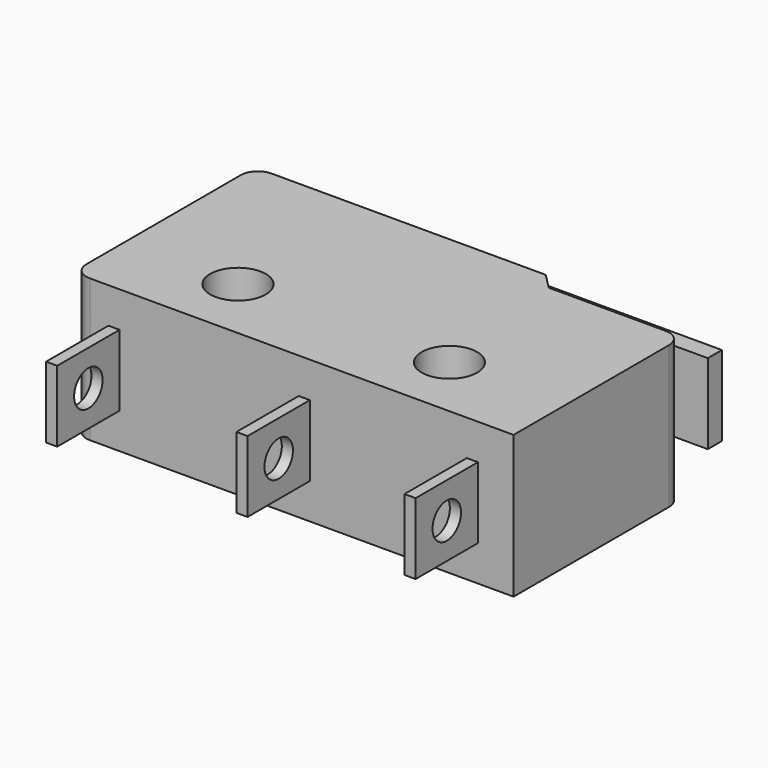
from build123d import *

# Parameters (mm, degrees)
F0_W     = 0.5
F0_H     = 3.5
F0_R     = 1.25
F1_DEPTH = 6.4
F2_W     = 1.5
F2_H     = 1.4
F2_W_2   = 3.5
F2_H_2   = 1.6
F2_R     = 0.8
F3_DEPTH = 19.8
F4_R     = 0.762


with BuildPart() as f1:
    # F0 (on Top) → F1 (new body)
    with BuildSketch(Plane.XY):
        with Locations((4.1668843009, -11.25)):
            Rectangle(F0_W, F0_H)
        with Locations((-3.3831156991, -11.25)):
            Rectangle(F0_W, F0_H)
        with Locations((-11.9331156991, -11.25)):
            Rectangle(F0_W, F0_H)
        with BuildLine():
            Line((-10.6081156991, 0.7), (-9.8143656991, 0.7))
            Line((-9.8143656991, 0.7), (-9.8143656991, 1.101979753))
            ThreePointArc((-9.8143656991, 1.101979753), (-9.7252470071, 1.317131308), (-9.5100954521, 1.40625))
            Line((-9.5100954521, 1.40625), (6.0168843009, 1.40625))
            Line((6.0168843009, 1.40625), (6.0168843009, 2.2))
            Line((6.0168843009, 2.2), (-9.5100954521, 2.2))
            ThreePointArc((-9.5100954521, 2.2), (-10.2865130147, 1.8783973155), (-10.6081156991, 1.101979753))
            Line((-10.6081156991, 1.101979753), (-10.6081156991, 0.7))
        make_face()
        with BuildLine():
            Line((6.0168843009, 0), (0, 0))
            Line((0, 0), (-0.7, 0.7))
            Line((-0.7, 0.7), (-5.9126656991, 0.7))
            ThreePointArc((-5.9126656991, 0.7), (-6.5935156991, 1.38085), (-7.2743656991, 0.7))
            Line((-7.2743656991, 0.7), (-9.8143656991, 0.7))
            Line((-9.8143656991, 0.7), (-10.6081156991, 0.7))
            Line((-10.6081156991, 0.7), (-13.7831156991, 0.7))
            Line((-13.7831156991, 0.7), (-13.7831156991, -9.5))
            Line((-13.7831156991, -9.5), (-12.1831156991, -9.5))
            Line((-12.1831156991, -9.5), (-11.6831156991, -9.5))
            Line((-11.6831156991, -9.5), (-3.6331156991, -9.5))
            Line((-3.6331156991, -9.5), (-3.1331156991, -9.5))
            Line((-3.1331156991, -9.5), (3.9168843009, -9.5))
            Line((3.9168843009, -9.5), (4.4168843009, -9.5))
            Line((4.4168843009, -9.5), (6.0168843009, -9.5))
            Line((6.0168843009, -9.5), (6.0168843009, 0))
        make_face()
        with Locations((-8.6831156991, -6.6)):
            Circle(F0_R, mode=Mode.SUBTRACT)
        with Locations((0.8168843009, -6.6)):
            Circle(F0_R, mode=Mode.SUBTRACT)
    extrude(amount=F1_DEPTH)

    # F2 (on face) → F3 (cut, through all)
    with BuildSketch(Plane(origin=(-13.7831156991, 0, 0), x_dir=(0, -1, 0), z_dir=(-1, 0, 0))):
        with Locations((-1.45, 0.7)):
            Rectangle(F2_W, F2_H)
        with Locations((-1.45, 5.7)):
            Rectangle(F2_W, F2_H)
        with Locations((11.25, 0.8)):
            Rectangle(F2_W_2, F2_H_2)
        with Locations((11.25, 5.6)):
            Rectangle(F2_W_2, F2_H_2)
        with Locations((11.25, 3.2)):
            Circle(F2_R)
    extrude(amount=-F3_DEPTH, mode=Mode.SUBTRACT)

    # F4
    f4_edges = [f1.edges().sort_by_distance(p)[0] for p in [
        (-13.783116, -9.5, 3.2),
        (6.016884, 0, 3.2),
        (-13.783116, 0.7, 3.2),
    ]]
    fillet(f4_edges, radius=F4_R)


solid = f1.part
